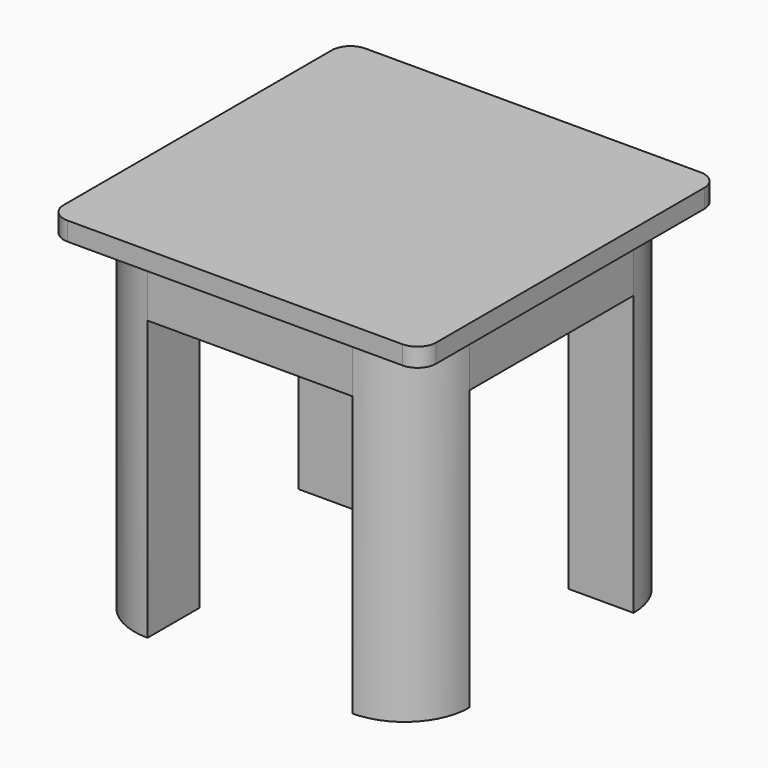
from build123d import *

# Parameters (mm, degrees)
F0_W     = 508
F0_H     = 508
F0_W_2   = 88.9
F0_H_2   = 88.9
F1_DEPTH = 25.4
F2_DEPTH = 101.6
F3_DEPTH = 482.6
F4_R     = 88.89999
F5_R     = 25.4


# Not quite as in the source:
# - a fillet or chamfer is up to 0.001 mm smaller than in the source, because OpenCascade refuses the exact size


with BuildPart() as f1:
    # F0 (on Top) → F1 (new body)
    with BuildSketch(Plane.XY):
        Rectangle(F0_W, F0_H)
        Polygon((139.7, 228.6), (228.6, 228.6), (228.6, 139.7), (228.6, -139.7), (228.6, -228.6), (139.7, -228.6), (-139.7, -228.6), (-228.6, -228.6), (-228.6, -139.7), (-228.6, 139.7), (-228.6, 228.6), (-139.7, 228.6), align=None, mode=Mode.SUBTRACT)
        with Locations((-184.15, -184.15)):
            Rectangle(F0_W_2, F0_H_2)
        with Locations((184.15, -184.15)):
            Rectangle(F0_W_2, F0_H_2)
        with Locations((184.15, 184.15)):
            Rectangle(F0_W_2, F0_H_2)
        with Locations((-184.15, 184.15)):
            Rectangle(F0_W_2, F0_H_2)
        Polygon((139.7, 139.7), (139.7, 228.6), (-139.7, 228.6), (-139.7, 139.7), (-228.6, 139.7), (-228.6, -139.7), (-139.7, -139.7), (-139.7, -228.6), (139.7, -228.6), (139.7, -139.7), (228.6, -139.7), (228.6, 139.7), align=None)
    extrude(amount=-F1_DEPTH)

    # F0 (on Top) → F2 (join)
    with BuildSketch(Plane.XY):
        with Locations((-184.15, 184.15)):
            Rectangle(F0_W_2, F0_H_2)
        Polygon((139.7, 139.7), (139.7, 228.6), (-139.7, 228.6), (-139.7, 139.7), (-228.6, 139.7), (-228.6, -139.7), (-139.7, -139.7), (-139.7, -228.6), (139.7, -228.6), (139.7, -139.7), (228.6, -139.7), (228.6, 139.7), align=None)
        with Locations((184.15, 184.15)):
            Rectangle(F0_W_2, F0_H_2)
        with Locations((184.15, -184.15)):
            Rectangle(F0_W_2, F0_H_2)
        with Locations((-184.15, -184.15)):
            Rectangle(F0_W_2, F0_H_2)
    extrude(amount=-F2_DEPTH)

    # F0 (on Top) → F3 (join)
    with BuildSketch(Plane.XY):
        with Locations((-184.15, 184.15)):
            Rectangle(F0_W_2, F0_H_2)
        with Locations((-184.15, -184.15)):
            Rectangle(F0_W_2, F0_H_2)
        with Locations((184.15, 184.15)):
            Rectangle(F0_W_2, F0_H_2)
        with Locations((184.15, -184.15)):
            Rectangle(F0_W_2, F0_H_2)
    extrude(amount=-F3_DEPTH)

    # F4 (radius 88.9 in the source; OpenCascade refuses exactly that, so slightly less here)
    f4_edges = [f1.edges().sort_by_distance(p)[0] for p in [
        (-228.6, -228.6, -254),
        (228.6, -228.6, -254),
        (228.6, 228.6, -254),
        (-228.6, 228.6, -254),
    ]]
    fillet(f4_edges, radius=F4_R)

    # F5
    f5_edges = [f1.edges().sort_by_distance(p)[0] for p in [
        (254, -254, -12.7),
        (254, 254, -12.7),
        (-254, 254, -12.7),
        (-254, -254, -12.7),
    ]]
    fillet(f5_edges, radius=F5_R)


solid = f1.part
